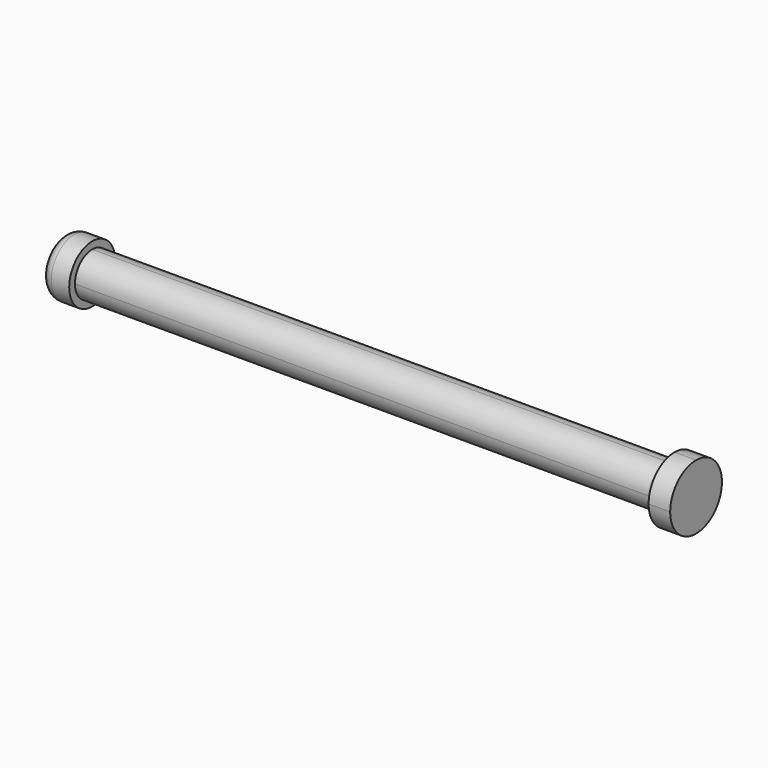
from build123d import *

# Parameters (mm, degrees)
F0_W     = 81
F0_H     = 6
F1_DEPTH = 3
F3_R     = 2.99999
F2_W     = 9
F2_H     = 9
F2_W_2   = 6
F2_H_2   = 6
F4_DEPTH = 3
F5_R     = 4.49999
F6_R     = 4
F7_DEPTH = 4
F8_R     = 1.5


# Not quite as in the source:
# - a fillet or chamfer is up to 0.001 mm smaller than in the source, because OpenCascade refuses the exact size
# - ends of sketch curves that miss each other by under 0.0002 mm in the source are joined


with BuildPart() as f1:
    # F0 (on Top) → F1 (new body, symmetric)
    with BuildSketch(Plane.XY):
        Rectangle(F0_W, F0_H)
    extrude(amount=F1_DEPTH, both=True)

    # F3 (radius 3 in the source; OpenCascade refuses exactly that, so slightly less here)
    f3_edges = [f1.edges().sort_by_distance(p)[0] for p in [
        (0, -3, 3),
        (0, -3, -3),
        (0, 3, 3),
        (0, 3, -3),
    ]]
    fillet(f3_edges, radius=F3_R)

    # F2 (on face) → F4 (join)
    with BuildSketch(Plane.YZ.offset(40.5)):
        Rectangle(F2_W, F2_H)
        Rectangle(F2_W_2, F2_H_2, mode=Mode.SUBTRACT)
        Rectangle(F2_W_2, F2_H_2)
    extrude(amount=F4_DEPTH)

    # F5 (radius 4.5 in the source; OpenCascade refuses exactly that, so slightly less here)
    f5_edges = [f1.edges().sort_by_distance(p)[0] for p in [
        (42, 4.5, 4.5),
        (42, -4.5, 4.5),
        (42, -4.5, -4.5),
        (42, 4.5, -4.5),
    ]]
    fillet(f5_edges, radius=F5_R)

    # F6 (on face) → F7 (join)
    with BuildSketch(Plane(origin=(-40.5, 0, 0), x_dir=(0, -1, 0), z_dir=(-1, 0, 0))):
        Circle(F6_R)
        with BuildLine():
            ThreePointArc((-1e-05, -3), (-2.1213232725, -2.1213232725), (-3, -1e-05))
            ThreePointArc((-3, -1e-05), (-2.1213232725, 2.1213232725), (-1e-05, 3))
            ThreePointArc((-1e-05, 3), (2.1213232725, 2.1213232725), (3, 1e-05))
            ThreePointArc((3, 1e-05), (2.1213232725, -2.1213232725), (-1e-05, -3))
        make_face(mode=Mode.SUBTRACT)
        with BuildLine():
            ThreePointArc((-1e-05, 3), (-2.1213232725, 2.1213232725), (-3, 1e-05))
            ThreePointArc((-3, 1e-05), (-2.1213232725, -2.1213232725), (-1e-05, -3))
            ThreePointArc((-1e-05, -3), (2.1213232725, -2.1213232725), (3, -1e-05))
            ThreePointArc((3, -1e-05), (2.1213232725, 2.1213232725), (-1e-05, 3))
        make_face()
    extrude(amount=F7_DEPTH)

    # F8
    f8_edges = [f1.edges().sort_by_distance(p)[0] for p in [
        (-44.5, 4, 0),
    ]]
    fillet(f8_edges, radius=F8_R)


solid = f1.part
